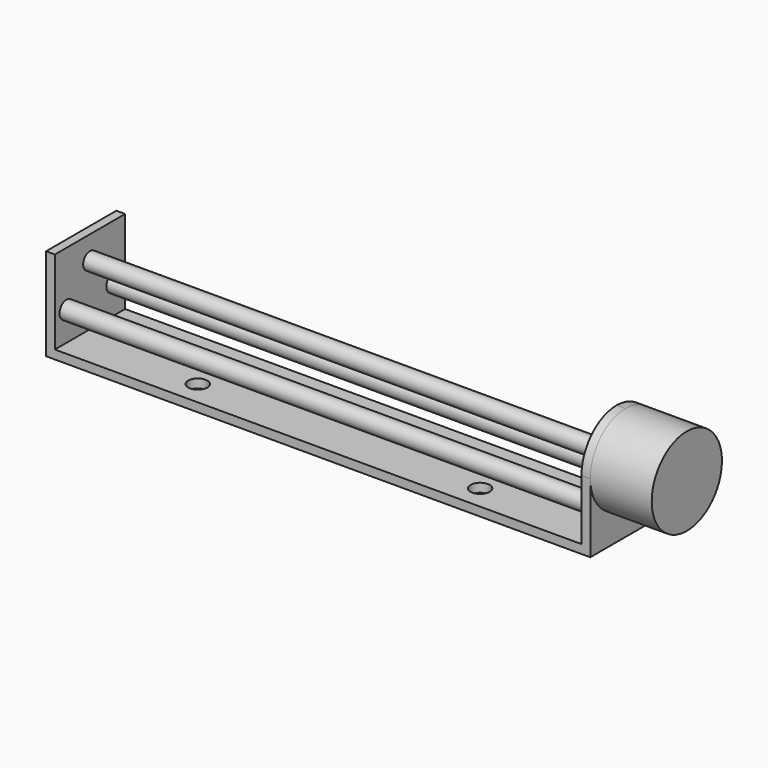
from build123d import *

# Parameters (mm, degrees)
F0_W      = 93
F0_H      = 15
F1_DEPTH  = 1.5
F2_W      = 1.5
F2_H      = 15
F3_DEPTH  = 14.3
F4_DEPTH  = 17.83
F6_DEPTH  = 10.5
F7_DEPTH  = 1.5
F8_R      = 1.5
F8_R_2    = 1.45
F9_DEPTH  = 90
F10_R     = 1.625
F11_DEPTH = 1.5


with BuildPart() as f1:
    # F0 (on Top) → F1 (new body)
    with BuildSketch(Plane.XY):
        with Locations((4.7561880201, -11.8954138505)):
            Rectangle(F0_W, F0_H)
    extrude(amount=F1_DEPTH)

    # F2 (on face) → F3 (join)
    with BuildSketch(Plane.XY.offset(1.5)):
        with Locations((-40.9938119799, -11.8954138505)):
            Rectangle(F2_W, F2_H)
    extrude(amount=F3_DEPTH)

    # F2 (on face) → F4 (join)
    with BuildSketch(Plane.XY.offset(1.5)):
        with Locations((50.5061880201, -11.8954138505)):
            Rectangle(F2_W, F2_H)
    extrude(amount=F4_DEPTH)

    # F5 (on face) → F6 (join)
    with BuildSketch(Plane.YZ.offset(51.2561880201)):
        with BuildLine():
            ThreePointArc((-19.3954138505, 11.83), (-11.8954138505, 4.33), (-4.3954138505, 11.83))
            ThreePointArc((-4.3954138505, 11.83), (-6.5921129916, 17.1333008589), (-11.8954138505, 19.33))
            ThreePointArc((-11.8954138505, 19.33), (-17.1987147094, 17.1333008589), (-19.3954138505, 11.83))
        make_face()
    extrude(amount=F6_DEPTH)

    # F7 (cut, through all): faces of the model
    f7_faces = [f1.faces().sort_by_distance(p)[0] for p in [
        (51.2561880201, -6.0706733926, 17.6547404579),
        (51.2561880201, -17.7201543084, 17.6547404579),
    ]]
    extrude(f7_faces, amount=-F7_DEPTH, mode=Mode.SUBTRACT)

    # F8 (on face) → F9 (join, through all)
    with BuildSketch(Plane(origin=(49.7561880201, 0, 0), x_dir=(0, -1, 0), z_dir=(-1, 0, 0))):
        with Locations((6.8954138505, 6.5)):
            Circle(F8_R)
        with Locations((11.8954138505, 11.83)):
            Circle(F8_R_2)
        with Locations((16.8954138505, 6.5)):
            Circle(F8_R)
    extrude(amount=F9_DEPTH)

    # F10 (on face) → F11 (cut, through all)
    with BuildSketch(Plane(origin=(0, 0, 0), x_dir=(1, 0, 0), z_dir=(0, 0, -1))):
        with Locations((-19.1188119799, 15.2704138505)):
            Circle(F10_R)
        with Locations((-19.1188119799, 8.5204138505)):
            Circle(F10_R)
        with Locations((29.1311880201, 8.5204138505)):
            Circle(F10_R)
        with Locations((29.1311880201, 15.2704138505)):
            Circle(F10_R)
    extrude(amount=-F11_DEPTH, mode=Mode.SUBTRACT)


solid = f1.part
